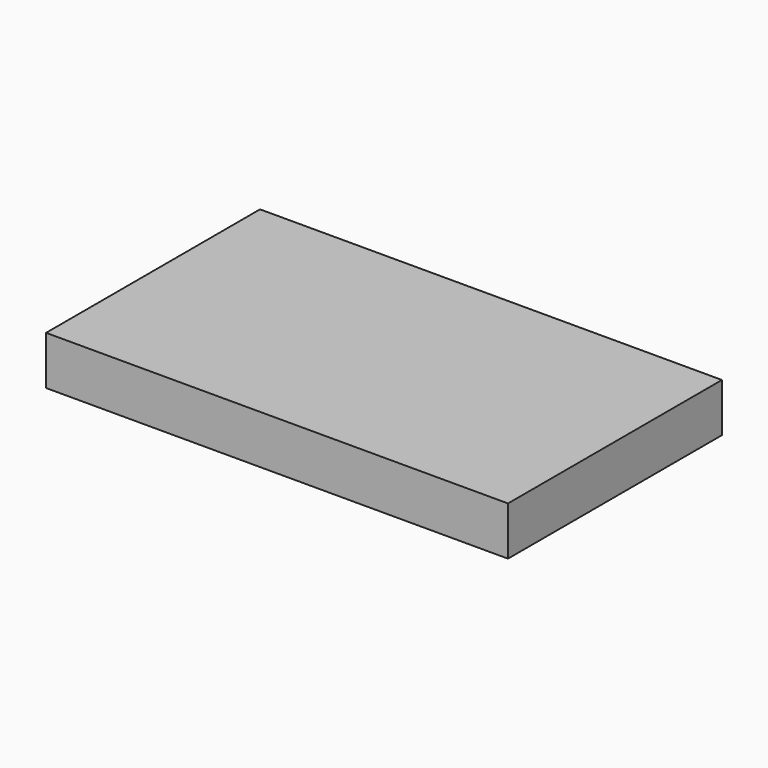
from build123d import *

# Parameters (mm, degrees)
F1_E0_BOTTOM_W = 95
F1_E0_BOTTOM_H = 55
F2_DEPTH       = 10


with BuildPart() as f2:
    # F1_E0_bottom (on explicit) → F2 (new body)
    with BuildSketch(Plane(origin=(-27.9861110127, 0, 0), x_dir=(1, 0, 0), z_dir=(0, 0, 1))):
        with Locations((47.5, 27.5)):
            Rectangle(F1_E0_BOTTOM_W, F1_E0_BOTTOM_H)
    extrude(amount=F2_DEPTH)


solid = f2.part
